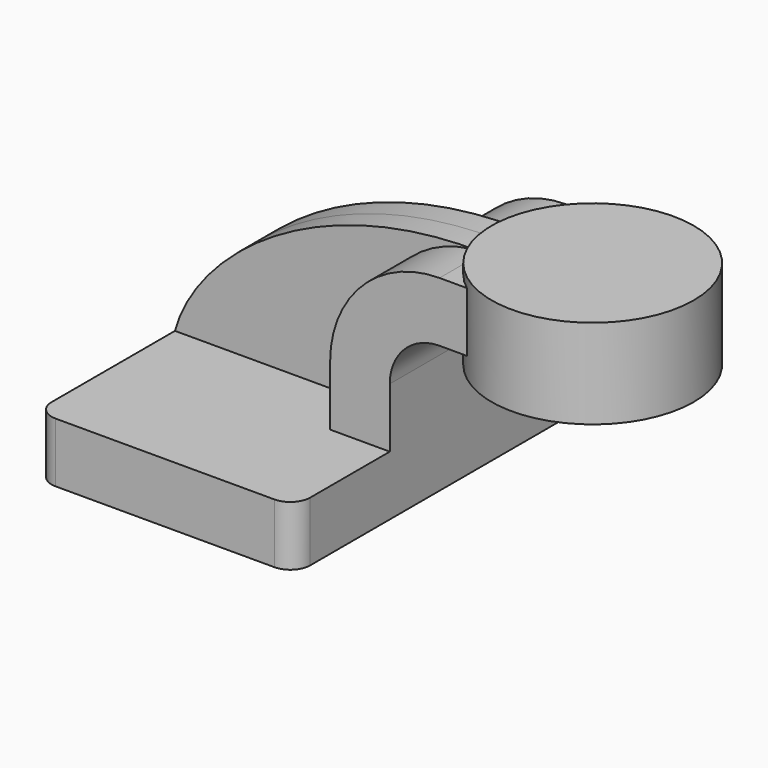
from build123d import *

# Parameters (mm, degrees)
F1_DEPTH = 63.5
F2_DEPTH = 25.4
F3_DEPTH = 7.9375
F5_R     = 6.35


# Not quite as in the source:
# - a feature names something its author has since deleted; it is built from what else it names


with BuildPart() as f1:
    # F0 (on Front) → F1 (new body, symmetric)
    with BuildSketch(Plane.XZ):
        Polygon((34.5979332924, 19.7320799329), (-28.9020667076, 19.7320799329), (-28.9020667076, 0.6820799329), (53.6479332924, 0.6820799329), (53.6479332924, 19.7320799329), align=None)
    extrude(amount=F1_DEPTH, both=True)

    # F0 (on Front) → F2 (join, symmetric)
    with BuildSketch(Plane.XZ):
        with BuildLine():
            Line((34.5979332924, 38.7820799329), (34.5979332924, 19.7320799329))
            Line((34.5979332924, 19.7320799329), (53.6479332924, 19.7320799329))
            Line((53.6479332924, 19.7320799329), (53.6479332924, 38.7820799329))
            ThreePointArc((53.6479332924, 38.7820799329), (58.2976131411, 50.0074000842), (69.5229332924, 54.6570799329))
            Line((69.5229332924, 54.6570799329), (79.5695575002, 54.6570799329))
            Line((79.5695575002, 54.6570799329), (79.5695575002, 73.7070799329))
            Line((79.5695575002, 73.7070799329), (69.5229332924, 73.7070799329))
            ThreePointArc((69.5229332924, 73.7070799329), (44.8272289594, 63.4777842658), (34.5979332924, 38.7820799329))
        make_face()
    extrude(amount=F2_DEPTH, both=True)

    # F0 (on Front) → F3 (join, symmetric)
    with BuildSketch(Plane.XZ):
        with BuildLine():
            add(Edge.make_bspline(
                [(-28.9020667076, 19.7320799329), (-21.9128355384, 45.4243458807), (16.2842553109, 74.7262239456), (69.5229332924, 73.7070799329)],
                knots=[0, 0, 0, 0, 112.2532015134, 112.2532015134, 112.2532015134, 112.2532015134], degree=3))
            Line((-28.9020667076, 19.7320799329), (34.5979332924, 19.7320799329))
            Line((34.5979332924, 19.7320799329), (34.5979332924, 38.7820799329))
            ThreePointArc((34.5979332924, 38.7820799329), (44.8272289594, 63.4777842658), (69.5229332924, 73.7070799329))
        make_face()
    extrude(amount=F3_DEPTH, both=True)

    # F5
    f5_edges = [f1.edges().sort_by_distance(p)[0] for p in [
        (-28.902067, -63.5, 10.20708),
        (53.647933, -63.5, 10.20708),
        (-28.902067, 63.5, 10.20708),
        (53.647933, 63.5, 10.20708),
    ]]
    fillet(f5_edges, radius=F5_R)


with BuildPart() as f4:
    # F0 (on Front) → F4 (revolve)
    with BuildSketch(Plane.XZ):
        Polygon((98.0979332924, 76.8820799329), (98.0979332924, 73.7070799329), (98.0979332924, 54.6570799329), (98.0979332924, 48.3070799329), (130.3695575002, 48.3070799329), (130.3695575002, 76.8820799329), align=None)
    revolve(axis=Axis((98.0979332924, 0, 62.5945799329), (0, 0, -1)))


solid = Compound([f1.part, f4.part])
